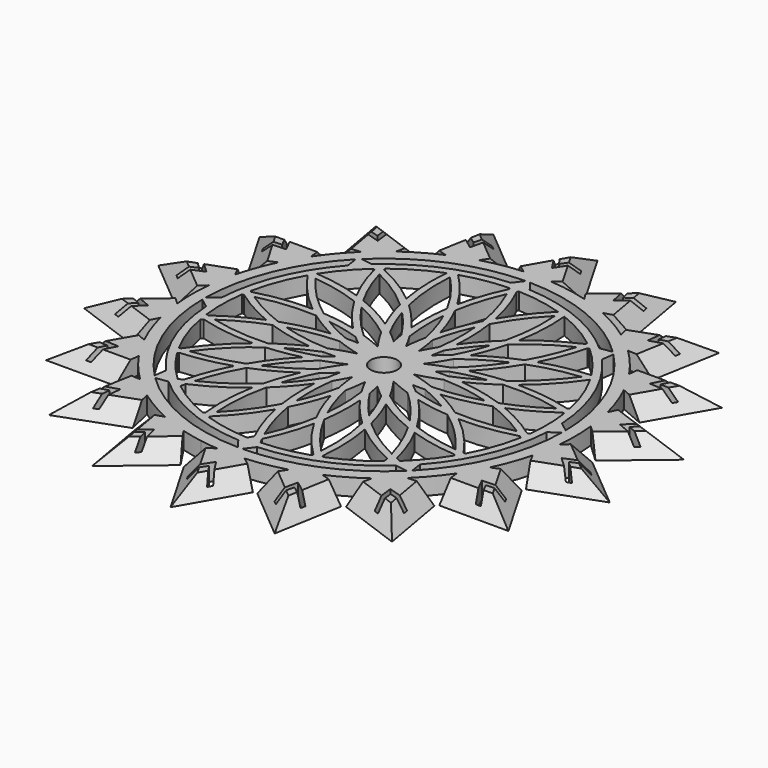
from build123d import *

# Parameters (mm, degrees)
F1_DEPTH      = 5.08
F2_T4_DEPTH   = 47.0360427955
F2_T9_DEPTH   = 47.0360427955
F2_T14_DEPTH  = 47.0360427955
F2_T19_DEPTH  = 47.0360427955
F2_T24_DEPTH  = 47.0360427955
F2_T29_DEPTH  = 47.0360427955
F2_T34_DEPTH  = 47.0360427955
F2_T39_DEPTH  = 47.0360427955
F2_T44_DEPTH  = 47.0360427955
F2_T49_DEPTH  = 47.0360427955
F2_T54_DEPTH  = 47.0360427955
F2_T59_DEPTH  = 47.0360427955
F2_T64_DEPTH  = 47.0360427955
F2_T69_DEPTH  = 47.0360427955
F2_T74_DEPTH  = 47.0360427955
F2_T79_DEPTH  = 47.0360427955
F2_T84_DEPTH  = 47.0360427955
F2_T89_DEPTH  = 47.0360427955
F2_T94_DEPTH  = 47.0360427955
F2_T99_DEPTH  = 47.0360427955
F2_T104_DEPTH = 47.0360427955
F2_T109_DEPTH = 47.0360427955
F2_T114_DEPTH = 47.0360427955
F2_T119_DEPTH = 47.0360427955
F2_T124_DEPTH = 47.0360427955
F2_T129_DEPTH = 47.0360427955
F2_T134_DEPTH = 47.0360427955
F2_T139_DEPTH = 47.0360427955
F2_T144_DEPTH = 47.0360427955
F2_T149_DEPTH = 47.0360427955
F2_T154_DEPTH = 47.0360427955
F2_T159_DEPTH = 47.0360427955
F2_T164_DEPTH = 47.0360427955
F2_T169_DEPTH = 47.0360427955
F2_T174_DEPTH = 47.0360427955
F2_T179_DEPTH = 47.0360427955
F4_DEPTH      = 5.08
F6_DEPTH      = 5.08
F7_R          = 55.2439698333
F7_R_2        = 49.2709923145
F8_DEPTH      = 5.08
F9_R          = 54.4459201536
F9_R_2        = 51.5980237821
F10_DEPTH     = 25.4
F12_DEPTH     = 5.08
F14_R         = 4.0270011847
F15_DEPTH     = 25.4


# Not quite as in the source:
# - a fillet or chamfer that OpenCascade refuses, or shapes differently, is made with other operations: its cross-section is extruded or revolved along the edge and cut away or added


with BuildPart() as f1:
    # F0 (on Top) → F1 (new body)
    with BuildSketch(Plane.XY):
        with BuildLine():
            ThreePointArc((15.9265090024, 55.862840854), (10.0864226386, 57.2064223286), (4.138989374, 57.941172272))
            Line((4.138989374, 57.941172272), (10.4434320733, 62.6353312958))
            Line((10.4434320733, 62.6353312958), (0, 80.7479918003))
            Line((0, 80.7479918003), (-10.4434320733, 62.6353312958))
            Line((-10.4434320733, 62.6353312958), (-4.140193851, 57.9410862184))
            ThreePointArc((-4.140193851, 57.9410862184), (-10.0876118404, 57.2062126403), (-15.9276702726, 55.8625097626))
            Line((-15.9276702726, 55.8625097626), (-11.6089289321, 62.4298227536))
            Line((-11.6089289321, 62.4298227536), (-27.6174397288, 75.878292038))
            Line((-27.6174397288, 75.878292038), (-31.236161042, 55.2860944846))
            Line((-31.236161042, 55.2860944846), (-23.7075282233, 53.0307814654))
            ThreePointArc((-23.7075282233, 53.0307814654), (-29.0449314541, 50.3060894337), (-34.073217817, 47.046004133))
            Line((-34.073217817, 47.046004133), (-32.2610817787, 54.6943562213))
            Line((-32.2610817787, 54.6943562213), (-51.9038086363, 61.8565504116))
            Line((-51.9038086363, 61.8565504116), (-48.2613479923, 41.2685387427))
            Line((-48.2613479923, 41.2685387427), (-40.415384806, 41.7241818167))
            ThreePointArc((-40.415384806, 41.7241818167), (-44.4990036769, 37.3383094027), (-48.1090324256, 32.5550560799))
            Line((-48.1090324256, 32.5550560799), (-49.02207204, 40.361943126))
            Line((-49.02207204, 40.361943126), (-69.9298122036, 40.3739959002))
            Line((-69.9298122036, 40.3739959002), (-59.4655041132, 22.2733881697))
            Line((-59.4655041132, 22.2733881697), (-52.2485495135, 25.3850300576))
            ThreePointArc((-52.2485495135, 25.3850300576), (-54.585839321, 19.8669782029), (-56.3421877099, 14.1374878021))
            Line((-56.3421877099, 14.1374878021), (-59.8702769245, 21.1612840109))
            Line((-59.8702769245, 21.1612840109), (-79.5212483651, 14.0217416264))
            Line((-79.5212483651, 14.0217416264), (-63.4972428207, 0.5917382633))
            Line((-63.4972428207, 0.5917382633), (-57.7797680432, 5.9840690304))
            ThreePointArc((-57.7797680432, 5.9840690304), (-58.0888171417, -0.0006037736), (-57.7796436342, -5.9852701517))
            Line((-57.7796436342, -5.9852701517), (-63.4972428207, -0.5917382633))
            Line((-63.4972428207, -0.5917382633), (-79.5212483651, -14.0217416264))
            Line((-79.5212483651, -14.0217416264), (-59.8702769245, -21.1612840109))
            Line((-59.8702769245, -21.1612840109), (-56.3418938084, -14.1386590373))
            ThreePointArc((-56.3418938084, -14.1386590373), (-54.5854263155, -19.868112926), (-52.2480217996, -25.3861161921))
            Line((-52.2480217996, -25.3861161921), (-59.4655041132, -22.2733881697))
            Line((-59.4655041132, -22.2733881697), (-69.9298122036, -40.3739959002))
            Line((-69.9298122036, -40.3739959002), (-49.02207204, -40.361943126))
            Line((-49.02207204, -40.361943126), (-48.1083556625, -32.5560561608))
            ThreePointArc((-48.1083556625, -32.5560561608), (-44.4982274806, -37.3392344374), (-40.4145174372, -41.7250219605))
            Line((-40.4145174372, -41.7250219605), (-48.2613479923, -41.2685387427))
            Line((-48.2613479923, -41.2685387427), (-51.9038086363, -61.8565504116))
            Line((-51.9038086363, -61.8565504116), (-32.2610817787, -54.6943562213))
            Line((-32.2610817787, -54.6943562213), (-34.0722398199, -47.046712435))
            ThreePointArc((-34.0722398199, -47.046712435), (-29.0438856876, -50.3066932073), (-23.7064258172, -53.0312742847))
            Line((-23.7064258172, -53.0312742847), (-31.236161042, -55.2860944846))
            Line((-31.236161042, -55.2860944846), (-27.6174397288, -75.878292038))
            Line((-27.6174397288, -75.878292038), (-11.6089289321, -62.4298227536))
            Line((-11.6089289321, -62.4298227536), (-15.9265090024, -55.862840854))
            ThreePointArc((-15.9265090024, -55.862840854), (-12.7601875814, -56.6699946195), (-9.5534900168, -57.2978315976))
            ThreePointArc((-9.5534900168, -57.2978315976), (-6.8578650316, -57.717343394), (-4.138989374, -57.941172272))
            Line((-4.138989374, -57.941172272), (-10.4434320733, -62.6353312958))
            Line((-10.4434320733, -62.6353312958), (0, -80.7479918003))
            Line((0, -80.7479918003), (10.4434320733, -62.6353312958))
            Line((10.4434320733, -62.6353312958), (4.140193851, -57.9410862184))
            ThreePointArc((4.140193851, -57.9410862184), (10.0876118404, -57.2062126403), (15.9276702726, -55.8625097626))
            Line((15.9276702726, -55.8625097626), (11.6089289321, -62.4298227536))
            Line((11.6089289321, -62.4298227536), (27.6174397288, -75.878292038))
            Line((27.6174397288, -75.878292038), (31.236161042, -55.2860944846))
            Line((31.236161042, -55.2860944846), (23.7075282233, -53.0307814654))
            ThreePointArc((23.7075282233, -53.0307814654), (29.0449314541, -50.3060894337), (34.073217817, -47.046004133))
            Line((34.073217817, -47.046004133), (32.2610817787, -54.6943562213))
            Line((32.2610817787, -54.6943562213), (51.9038086363, -61.8565504116))
            Line((51.9038086363, -61.8565504116), (48.2613479923, -41.2685387427))
            Line((48.2613479923, -41.2685387427), (40.415384806, -41.7241818167))
            ThreePointArc((40.415384806, -41.7241818167), (44.4990036769, -37.3383094027), (48.1090324256, -32.5550560799))
            Line((48.1090324256, -32.5550560799), (49.02207204, -40.361943126))
            Line((49.02207204, -40.361943126), (69.9298122036, -40.3739959002))
            Line((69.9298122036, -40.3739959002), (59.4655041132, -22.2733881697))
            Line((59.4655041132, -22.2733881697), (52.2485495135, -25.3850300576))
            ThreePointArc((52.2485495135, -25.3850300576), (54.585839321, -19.8669782029), (56.3421877099, -14.1374878021))
            Line((56.3421877099, -14.1374878021), (59.8702769245, -21.1612840109))
            Line((59.8702769245, -21.1612840109), (79.5212483651, -14.0217416264))
            Line((79.5212483651, -14.0217416264), (63.4972428207, -0.5917382633))
            Line((63.4972428207, -0.5917382633), (57.7797680432, -5.9840690304))
            ThreePointArc((57.7797680432, -5.9840690304), (58.0888171417, 0.0006037736), (57.7796436342, 5.9852701517))
            Line((57.7796436342, 5.9852701517), (63.4972428207, 0.5917382633))
            Line((63.4972428207, 0.5917382633), (79.5212483651, 14.0217416264))
            Line((79.5212483651, 14.0217416264), (59.8702769245, 21.1612840109))
            Line((59.8702769245, 21.1612840109), (56.3418938084, 14.1386590373))
            ThreePointArc((56.3418938084, 14.1386590373), (54.5854263155, 19.868112926), (52.2480217996, 25.3861161921))
            Line((52.2480217996, 25.3861161921), (59.4655041132, 22.2733881697))
            Line((59.4655041132, 22.2733881697), (69.9298122036, 40.3739959002))
            Line((69.9298122036, 40.3739959002), (49.02207204, 40.361943126))
            Line((49.02207204, 40.361943126), (48.1083556625, 32.5560561608))
            ThreePointArc((48.1083556625, 32.5560561608), (44.4982274806, 37.3392344374), (40.4145174372, 41.7250219605))
            Line((40.4145174372, 41.7250219605), (48.2613479923, 41.2685387427))
            Line((48.2613479923, 41.2685387427), (51.9038086363, 61.8565504116))
            Line((51.9038086363, 61.8565504116), (32.2610817787, 54.6943562213))
            Line((32.2610817787, 54.6943562213), (34.0722398199, 47.046712435))
            ThreePointArc((34.0722398199, 47.046712435), (29.0438856876, 50.3066932073), (23.7064258172, 53.0312742847))
            Line((23.7064258172, 53.0312742847), (31.236161042, 55.2860944846))
            Line((31.236161042, 55.2860944846), (27.6174397288, 75.878292038))
            Line((27.6174397288, 75.878292038), (11.6089289321, 62.4298227536))
            Line((11.6089289321, 62.4298227536), (15.9265090024, 55.862840854))
        make_face()
        Polygon((-40.8170132151, -48.6438221381), (-41.6786948496, -55.6460012024), (-43.1171047598, -56.1704788463), (-42.4937358465, -50.6420623579), (-47.8299146071, -52.2159618416), (-47.5631825433, -50.708329749), align=None, mode=Mode.SUBTRACT)
        Polygon((-21.7182791012, -59.6704814199), (-20.1331086874, -66.5450898922), (-21.3053899468, -67.5299028276), (-22.6104445787, -62.1216859237), (-27.0865070562, -65.425748279), (-27.3515014484, -63.917809788), align=None, mode=Mode.SUBTRACT)
        Polygon((-54.9926131403, -31.75), (-58.1972153009, -38.03518352), (-59.7282603981, -38.0360661281), (-57.2516554306, -33.0542586744), (-62.8043285621, -32.7081597806), (-62.0380418656, -31.382676767), align=None, mode=Mode.SUBTRACT)
        Polygon((-62.5352923163, -11.0266592818), (-67.6962926875, -15.8367613656), (-69.1353063372, -15.3139424824), (-65.1041804252, -11.4796235659), (-70.2036135993, -9.255270929), (-69.0301977549, -8.271809808), align=None, mode=Mode.SUBTRACT)
        Polygon((3.0760693279, -70.7442238927), (0, -66.1085173488), (-3.076067, -70.7442238927), (-3.8408256137, -69.4178586401), (0, -63.5), (3.8408275155, -69.4178586401), align=None, mode=Mode.SUBTRACT)
        Polygon((27.0865092437, -65.4257474828), (22.6104445787, -62.1216859237), (21.3053921343, -67.5299020314), (20.1331104745, -66.5450892418), (21.7182791012, -59.6704814199), (27.3515032355, -63.9178091375), align=None, mode=Mode.SUBTRACT)
        Polygon((47.8299163904, -52.2159603452), (42.4937358465, -50.6420623579), (43.1171065431, -56.1704773499), (41.6786963064, -55.64599998), (40.8170132151, -48.6438221381), (47.563184, -50.7083285266), align=None, mode=Mode.SUBTRACT)
        with BuildLine():
            ThreePointArc((53.4287791534, 0), (-37.7798520499, -37.7798520499), (0, 53.4287791534))
            ThreePointArc((0, 53.4287791534), (37.7798520499, 37.7798520499), (53.4287791534, 0))
        make_face(mode=Mode.SUBTRACT)
        Polygon((62.804329726, -32.7081577646), (57.2516554306, -33.0542586744), (59.7282615621, -38.0360641121), (58.1972162518, -38.0351818731), (54.9926131403, -31.75), (62.0380428164, -31.3826751201), align=None, mode=Mode.SUBTRACT)
        Polygon((70.2036140035, -9.2552686365), (65.1041804252, -11.4796235659), (69.1353067414, -15.3139401898), (67.6962930177, -15.8367594928), (62.5352923163, -11.0266592819), (69.0301980851, -8.2718079352), align=None, mode=Mode.SUBTRACT)
        Polygon((-62.5352923163, 11.0266592819), (-69.0301980851, 8.2718079352), (-70.2036140035, 9.2552686365), (-65.1041804252, 11.4796235659), (-69.1353067414, 15.3139401898), (-67.6962930177, 15.8367594928), align=None, mode=Mode.SUBTRACT)
        Polygon((-54.9926131403, 31.75), (-62.0380428164, 31.3826751201), (-62.804329726, 32.7081577646), (-57.2516554306, 33.0542586744), (-59.7282615621, 38.0360641121), (-58.1972162518, 38.0351818731), align=None, mode=Mode.SUBTRACT)
        Polygon((-40.8170132151, 48.6438221381), (-47.563184, 50.7083285266), (-47.8299163904, 52.2159603452), (-42.4937358465, 50.6420623579), (-43.1171065431, 56.1704773499), (-41.6786963064, 55.64599998), align=None, mode=Mode.SUBTRACT)
        Polygon((-21.7182791012, 59.6704814199), (-27.3515032355, 63.9178091376), (-27.0865092437, 65.4257474828), (-22.6104445787, 62.1216859237), (-21.3053921343, 67.5299020314), (-20.1331104745, 66.5450892418), align=None, mode=Mode.SUBTRACT)
        Polygon((3.8408256138, 69.4178586401), (0, 63.5), (-3.8408275155, 69.4178586401), (-3.0760693279, 70.7442238927), (0, 66.1085173488), (3.076067, 70.7442238927), align=None, mode=Mode.SUBTRACT)
        Polygon((69.1353063372, 15.3139424824), (65.1041804252, 11.4796235659), (70.2036135993, 9.255270929), (69.0301977548, 8.271809808), (62.5352923163, 11.0266592818), (67.6962926875, 15.8367613656), align=None, mode=Mode.SUBTRACT)
        Polygon((59.7282603981, 38.0360661281), (57.2516554306, 33.0542586744), (62.8043285621, 32.7081597806), (62.0380418655, 31.382676767), (54.9926131403, 31.75), (58.1972153009, 38.03518352), align=None, mode=Mode.SUBTRACT)
        Polygon((21.3053899468, 67.5299028276), (22.6104445787, 62.1216859237), (27.0865070562, 65.425748279), (27.3515014484, 63.917809788), (21.7182791012, 59.6704814199), (20.1331086874, 66.5450898922), align=None, mode=Mode.SUBTRACT)
        Polygon((43.1171047598, 56.1704788463), (42.4937358465, 50.6420623579), (47.8299146071, 52.2159618416), (47.5631825432, 50.708329749), (40.8170132151, 48.6438221381), (41.6786948496, 55.6460012024), align=None, mode=Mode.SUBTRACT)
    extrude(amount=F1_DEPTH)

    # F2: chamfer of 5.08 on 36 edges, made by hand


with BuildPart() as f2_tool2:
    # F2_s3 → F2_t4 (new body)
    with BuildSketch(Plane(origin=(-6.2684927358, -35.4309391934, 0), x_dir=(0, 0, 1), z_dir=(-0.174215865, -0.9847074857, 0))):
        Polygon((5.08, 35.2536764612), (0, 40.3336764612), (5.08, 40.3336764612), align=None)
    extrude(amount=F2_T4_DEPTH)

    split(bisect_by=Plane(origin=(-2.5554446187, -43.9274438504, 0), x_dir=(0, 0, 1), z_dir=(-0.0580760277, -0.9983121631, 0)), keep=Keep.TOP)


with BuildPart() as f1_1:
    add(f1.part)

    # F2_t1: cut F2_tool2
    add(f2_tool2.part, mode=Mode.SUBTRACT)


with BuildPart() as f2_tool7:
    # F2_s8 → F2_t9 (new body)
    with BuildSketch(Plane(origin=(-77.9942923576, -28.4385295204, 0), x_dir=(0, 0, 1), z_dir=(0.9394952989, 0.342561795, 0))):
        Polygon((5.08, 35.2536764612), (0, 40.3336764612), (5.08, 40.3336764612), align=None)
    extrude(amount=F2_T9_DEPTH)

    split(bisect_by=Plane(origin=(-42.8128872524, -10.1391889033, 0), x_dir=(0, 0, 1), z_dir=(-0.9730838832, -0.2304512016, 0)), keep=Keep.TOP)


with BuildPart() as f1_2:
    add(f1_1.part)

    # F2_t6: cut F2_tool7
    add(f2_tool7.part, mode=Mode.SUBTRACT)


with BuildPart() as f2_tool12:
    # F2_s13 → F2_t14 (new body)
    with BuildSketch(Plane(origin=(6.2276385338, -35.4381428915, 0), x_dir=(0, 0, 1), z_dir=(0.1730804326, -0.9849076931, 0))):
        Polygon((5.08, 35.2536764612), (0, 40.3336764612), (5.08, 40.3336764612), align=None)
    extrude(amount=F2_T14_DEPTH)

    split(bisect_by=Plane(origin=(12.6227381906, -42.1523083709, 0), x_dir=(0, 0, 1), z_dir=(0.2868692545, -0.9579697442, 0)), keep=Keep.TOP)


with BuildPart() as f1_3:
    add(f1_2.part)

    # F2_t11: cut F2_tool12
    add(f2_tool12.part, mode=Mode.SUBTRACT)


with BuildPart() as f2_tool17:
    # F2_s18 → F2_t19 (new body)
    with BuildSketch(Plane(origin=(-63.5641110493, -53.399095387, 0), x_dir=(0, 0, 1), z_dir=(0.7656737654, 0.6432291077, 0))):
        Polygon((5.08, 35.2536764612), (0, 40.3336764612), (5.08, 40.3336764612), align=None)
    extrude(amount=F2_T19_DEPTH)

    split(bisect_by=Plane(origin=(-36.7631473837, -24.1705908274, 0), x_dir=(0, 0, 1), z_dir=(-0.8355807914, -0.5493675828, 0)), keep=Keep.TOP)


with BuildPart() as f1_4:
    add(f1_3.part)

    # F2_t16: cut F2_tool17
    add(f2_tool17.part, mode=Mode.SUBTRACT)


with BuildPart() as f2_tool22:
    # F2_s23 → F2_t24 (new body)
    with BuildSketch(Plane(origin=(17.9726246861, -31.1709835456, 0), x_dir=(0, 0, 1), z_dir=(0.4995006756, -0.866313497, 0))):
        Polygon((5.08, 35.2536764612), (0, 40.3336764612), (5.08, 40.3336764612), align=None)
    extrude(amount=F2_T24_DEPTH)

    split(bisect_by=Plane(origin=(26.2784324824, -35.2929824001, 0), x_dir=(0, 0, 1), z_dir=(0.5972138708, -0.8020820361, 0)), keep=Keep.TOP)


with BuildPart() as f1_5:
    add(f1_4.part)

    # F2_t21: cut F2_tool22
    add(f2_tool22.part, mode=Mode.SUBTRACT)


with BuildPart() as f2_tool27:
    # F2_s28 → F2_t29 (new body)
    with BuildSketch(Plane(origin=(-41.4671598421, -71.9189422632, 0), x_dir=(0, 0, 1), z_dir=(0.4995006756, 0.866313497, 0))):
        Polygon((5.08, 35.2536764613), (0, 40.3336764613), (5.08, 40.3336764613), align=None)
    extrude(amount=F2_T29_DEPTH)

    split(bisect_by=Plane(origin=(-26.2792293743, -35.2866627778, 0), x_dir=(0, 0, 1), z_dir=(-0.5972943244, -0.8020221257, 0)), keep=Keep.TOP)


with BuildPart() as f1_6:
    add(f1_5.part)

    # F2_t26: cut F2_tool27
    add(f2_tool27.part, mode=Mode.SUBTRACT)


with BuildPart() as f2_tool32:
    # F2_s33 → F2_t34 (new body)
    with BuildSketch(Plane(origin=(27.5498470535, -23.1441435493, 0), x_dir=(0, 0, 1), z_dir=(0.7656737654, -0.6432291077, 0))):
        Polygon((5.08, 35.2536764612), (0, 40.3336764612), (5.08, 40.3336764612), align=None)
    extrude(amount=F2_T34_DEPTH)

    split(bisect_by=Plane(origin=(36.7645599884, -24.1768018828, 0), x_dir=(0, 0, 1), z_dir=(0.8355256803, -0.5494513969, 0)), keep=Keep.TOP)


with BuildPart() as f1_7:
    add(f1_6.part)

    # F2_t31: cut F2_tool32
    add(f2_tool32.part, mode=Mode.SUBTRACT)


with BuildPart() as f2_tool37:
    # F2_s38 → F2_t39 (new body)
    with BuildSketch(Plane(origin=(-14.3686571678, -81.7643032921, 0), x_dir=(0, 0, 1), z_dir=(0.1730804326, 0.9849076931, 0))):
        Polygon((5.08, 35.2536764612), (0, 40.3336764612), (5.08, 40.3336764612), align=None)
    extrude(amount=F2_T39_DEPTH)

    split(bisect_by=Plane(origin=(-12.6256484622, -42.1466424216, 0), x_dir=(0, 0, 1), z_dir=(-0.2869653467, -0.9579409636, 0)), keep=Keep.TOP)


with BuildPart() as f1_8:
    add(f1_7.part)

    # F2_t36: cut F2_tool37
    add(f2_tool37.part, mode=Mode.SUBTRACT)


with BuildPart() as f2_tool42:
    # F2_s43 → F2_t44 (new body)
    with BuildSketch(Plane(origin=(33.8041512739, -12.3257782699, 0), x_dir=(0, 0, 1), z_dir=(0.9394952989, -0.342561795, 0))):
        Polygon((5.08, 35.2536764612), (0, 40.3336764612), (5.08, 40.3336764612), align=None)
    extrude(amount=F2_T44_DEPTH)

    split(bisect_by=Plane(origin=(42.8163389727, -10.144542247, 0), x_dir=(0, 0, 1), z_dir=(0.9730607618, -0.2305488102, 0)), keep=Keep.TOP)


with BuildPart() as f1_9:
    add(f1_8.part)

    # F2_t41: cut F2_tool42
    add(f2_tool42.part, mode=Mode.SUBTRACT)


with BuildPart() as f2_tool47:
    # F2_s48 → F2_t49 (new body)
    with BuildSketch(Plane(origin=(14.4629176196, -81.7476826312, 0), x_dir=(0, 0, 1), z_dir=(-0.174215865, 0.9847074857, 0))):
        Polygon((5.08, 35.2536764612), (0, 40.3336764612), (5.08, 40.3336764612), align=None)
    extrude(amount=F2_T49_DEPTH)

    split(bisect_by=Plane(origin=(2.5507719892, -43.9231149711, 0), x_dir=(0, 0, 1), z_dir=(0.057975887, -0.9983179837, 0)), keep=Keep.TOP)


with BuildPart() as f1_10:
    add(f1_9.part)

    # F2_t46: cut F2_tool47
    add(f2_tool47.part, mode=Mode.SUBTRACT)


with BuildPart() as f2_tool52:
    # F2_s53 → F2_t54 (new body)
    with BuildSketch(Plane(origin=(35.9811759544, -0.0207422219, 0), x_dir=(0, 0, 1), z_dir=(0.9999998338, -0.0005764742, 0))):
        Polygon((5.08, 35.2536764612), (0, 40.3336764612), (5.08, 40.3336764612), align=None)
    extrude(amount=F2_T54_DEPTH)

    split(bisect_by=Plane(origin=(43.703835575, 5.1112989013, 0), x_dir=(0, 0, 1), z_dir=(0.9932303545, 0.1161613655, 0)), keep=Keep.TOP)


with BuildPart() as f1_11:
    add(f1_10.part)

    # F2_t51: cut F2_tool52
    add(f2_tool52.part, mode=Mode.SUBTRACT)


with BuildPart() as f2_tool57:
    # F2_s58 → F2_t59 (new body)
    with BuildSketch(Plane(origin=(41.5500510922, -71.8710849777, 0), x_dir=(0, 0, 1), z_dir=(-0.5004991582, 0.8657370228, 0))):
        Polygon((5.08, 35.2536764612), (0, 40.3336764612), (5.08, 40.3336764612), align=None)
    extrude(amount=F2_T59_DEPTH)

    split(bisect_by=Plane(origin=(17.4195316933, -40.401811619, 0), x_dir=(0, 0, 1), z_dir=(0.395924373, -0.9182831213, 0)), keep=Keep.TOP)


with BuildPart() as f1_12:
    add(f1_11.part)

    # F2_t56: cut F2_tool57
    add(f2_tool57.part, mode=Mode.SUBTRACT)


with BuildPart() as f2_tool62:
    # F2_s63 → F2_t64 (new body)
    with BuildSketch(Plane(origin=(33.8183397893, 12.2867956441, 0), x_dir=(0, 0, 1), z_dir=(0.9398896304, 0.341478378, 0))):
        Polygon((5.08, 35.2536764612), (0, 40.3336764612), (5.08, 40.3336764612), align=None)
    extrude(amount=F2_T64_DEPTH)

    split(bisect_by=Plane(origin=(39.3200046071, 19.7506419674, 0), x_dir=(0, 0, 1), z_dir=(0.893601708, 0.4488607662, 0)), keep=Keep.TOP)


with BuildPart() as f1_13:
    add(f1_12.part)

    # F2_t61: cut F2_tool62
    add(f2_tool62.part, mode=Mode.SUBTRACT)


with BuildPart() as f2_tool67:
    # F2_s68 → F2_t69 (new body)
    with BuildSketch(Plane(origin=(63.6256351897, -53.3257737717, 0), x_dir=(0, 0, 1), z_dir=(-0.7664148663, 0.642345898, 0))):
        Polygon((5.08, 35.2536764612), (0, 40.3336764612), (5.08, 40.3336764612), align=None)
    extrude(amount=F2_T69_DEPTH)

    split(bisect_by=Plane(origin=(30.1872387902, -32.0074535183, 0), x_dir=(0, 0, 1), z_dir=(0.6861185365, -0.7274897621, 0)), keep=Keep.TOP)


with BuildPart() as f1_14:
    add(f1_13.part)

    # F2_t66: cut F2_tool67
    add(f2_tool67.part, mode=Mode.SUBTRACT)


with BuildPart() as f2_tool72:
    # F2_s73 → F2_t74 (new body)
    with BuildSketch(Plane(origin=(27.57651274, 23.1123646216, 0), x_dir=(0, 0, 1), z_dir=(0.7664148663, 0.642345898, 0))):
        Polygon((5.08, 35.2536764612), (0, 40.3336764612), (5.08, 40.3336764612), align=None)
    extrude(amount=F2_T74_DEPTH)

    split(bisect_by=Plane(origin=(30.193600782, 32.0077661239, 0), x_dir=(0, 0, 1), z_dir=(0.6861915073, 0.727420934, 0)), keep=Keep.TOP)


with BuildPart() as f1_15:
    add(f1_14.part)

    # F2_t71: cut F2_tool72
    add(f2_tool72.part, mode=Mode.SUBTRACT)


with BuildPart() as f2_tool77:
    # F2_s78 → F2_t79 (new body)
    with BuildSketch(Plane(origin=(78.0270286689, -28.3485872441, 0), x_dir=(0, 0, 1), z_dir=(-0.9398896304, 0.341478378, 0))):
        Polygon((5.08, 35.2536764612), (0, 40.3336764612), (5.08, 40.3336764612), align=None)
    extrude(amount=F2_T79_DEPTH)

    split(bisect_by=Plane(origin=(39.3139193729, -19.7525241437, 0), x_dir=(0, 0, 1), z_dir=(0.8935566784, -0.4489504009, 0)), keep=Keep.TOP)


with BuildPart() as f1_16:
    add(f1_15.part)

    # F2_t76: cut F2_tool77
    add(f2_tool77.part, mode=Mode.SUBTRACT)


with BuildPart() as f2_tool82:
    # F2_s83 → F2_t84 (new body)
    with BuildSketch(Plane(origin=(41.4671598421, 71.9189422633, 0), x_dir=(0, 0, 1), z_dir=(-0.4995006756, -0.866313497, 0))):
        Polygon((5.08, 35.2536764612), (0, 40.3336764612), (5.08, 40.3336764612), align=None)
    extrude(amount=F2_T84_DEPTH)

    split(bisect_by=Plane(origin=(26.2792293743, 35.2866627779, 0), x_dir=(0, 0, 1), z_dir=(0.5972943244, 0.8020221257, 0)), keep=Keep.TOP)


with BuildPart() as f1_17:
    add(f1_16.part)

    # F2_t81: cut F2_tool82
    add(f2_tool82.part, mode=Mode.SUBTRACT)


with BuildPart() as f2_tool87:
    # F2_s88 → F2_t89 (new body)
    with BuildSketch(Plane(origin=(-27.5498470535, 23.1441435493, 0), x_dir=(0, 0, 1), z_dir=(-0.7656737654, 0.6432291077, 0))):
        Polygon((5.08, 35.2536764612), (0, 40.3336764612), (5.08, 40.3336764612), align=None)
    extrude(amount=F2_T89_DEPTH)

    split(bisect_by=Plane(origin=(-36.7645599884, 24.1768018829, 0), x_dir=(0, 0, 1), z_dir=(-0.8355256803, 0.5494513969, 0)), keep=Keep.TOP)


with BuildPart() as f1_18:
    add(f1_17.part)

    # F2_t86: cut F2_tool87
    add(f2_tool87.part, mode=Mode.SUBTRACT)


with BuildPart() as f2_tool92:
    # F2_s93 → F2_t94 (new body)
    with BuildSketch(Plane(origin=(14.3686571679, 81.764303292, 0), x_dir=(0, 0, 1), z_dir=(-0.1730804326, -0.9849076931, 0))):
        Polygon((5.08, 35.2536764612), (0, 40.3336764612), (5.08, 40.3336764612), align=None)
    extrude(amount=F2_T94_DEPTH)

    split(bisect_by=Plane(origin=(12.6256484622, 42.1466424216, 0), x_dir=(0, 0, 1), z_dir=(0.2869653467, 0.9579409636, 0)), keep=Keep.TOP)


with BuildPart() as f1_19:
    add(f1_18.part)

    # F2_t91: cut F2_tool92
    add(f2_tool92.part, mode=Mode.SUBTRACT)


with BuildPart() as f2_tool97:
    # F2_s98 → F2_t99 (new body)
    with BuildSketch(Plane(origin=(-33.8041512739, 12.3257782699, 0), x_dir=(0, 0, 1), z_dir=(-0.9394952989, 0.342561795, 0))):
        Polygon((5.08, 35.2536764612), (0, 40.3336764612), (5.08, 40.3336764612), align=None)
    extrude(amount=F2_T99_DEPTH)

    split(bisect_by=Plane(origin=(-42.8163389727, 10.144542247, 0), x_dir=(0, 0, 1), z_dir=(-0.9730607618, 0.2305488102, 0)), keep=Keep.TOP)


with BuildPart() as f1_20:
    add(f1_19.part)

    # F2_t96: cut F2_tool97
    add(f2_tool97.part, mode=Mode.SUBTRACT)


with BuildPart() as f2_tool102:
    # F2_s103 → F2_t104 (new body)
    with BuildSketch(Plane(origin=(-14.4629176196, 81.7476826312, 0), x_dir=(0, 0, 1), z_dir=(0.174215865, -0.9847074857, 0))):
        Polygon((5.08, 35.2536764612), (0, 40.3336764612), (5.08, 40.3336764612), align=None)
    extrude(amount=F2_T104_DEPTH)

    split(bisect_by=Plane(origin=(-2.5507719892, 43.9231149711, 0), x_dir=(0, 0, 1), z_dir=(-0.057975887, 0.9983179837, 0)), keep=Keep.TOP)


with BuildPart() as f1_21:
    add(f1_20.part)

    # F2_t101: cut F2_tool102
    add(f2_tool102.part, mode=Mode.SUBTRACT)


with BuildPart() as f2_tool107:
    # F2_s108 → F2_t109 (new body)
    with BuildSketch(Plane(origin=(-35.9811759544, 0.0207422219, 0), x_dir=(0, 0, 1), z_dir=(-0.9999998338, 0.0005764742, 0))):
        Polygon((5.08, 35.2536764612), (0, 40.3336764612), (5.08, 40.3336764612), align=None)
    extrude(amount=F2_T109_DEPTH)

    split(bisect_by=Plane(origin=(-43.703835575, -5.1112989013, 0), x_dir=(0, 0, 1), z_dir=(-0.9932303545, -0.1161613655, 0)), keep=Keep.TOP)


with BuildPart() as f1_22:
    add(f1_21.part)

    # F2_t106: cut F2_tool107
    add(f2_tool107.part, mode=Mode.SUBTRACT)


with BuildPart() as f2_tool112:
    # F2_s113 → F2_t114 (new body)
    with BuildSketch(Plane(origin=(-41.5500510923, 71.8710849777, 0), x_dir=(0, 0, 1), z_dir=(0.5004991582, -0.8657370228, 0))):
        Polygon((5.08, 35.2536764612), (0, 40.3336764612), (5.08, 40.3336764612), align=None)
    extrude(amount=F2_T114_DEPTH)

    split(bisect_by=Plane(origin=(-17.4195316933, 40.401811619, 0), x_dir=(0, 0, 1), z_dir=(-0.395924373, 0.9182831213, 0)), keep=Keep.TOP)


with BuildPart() as f1_23:
    add(f1_22.part)

    # F2_t111: cut F2_tool112
    add(f2_tool112.part, mode=Mode.SUBTRACT)


with BuildPart() as f2_tool117:
    # F2_s118 → F2_t119 (new body)
    with BuildSketch(Plane(origin=(-33.8183397893, -12.2867956441, 0), x_dir=(0, 0, 1), z_dir=(-0.9398896304, -0.341478378, 0))):
        Polygon((5.08, 35.2536764612), (0, 40.3336764612), (5.08, 40.3336764612), align=None)
    extrude(amount=F2_T119_DEPTH)

    split(bisect_by=Plane(origin=(-39.320004607, -19.7506419675, 0), x_dir=(0, 0, 1), z_dir=(-0.893601708, -0.4488607662, 0)), keep=Keep.TOP)


with BuildPart() as f1_24:
    add(f1_23.part)

    # F2_t116: cut F2_tool117
    add(f2_tool117.part, mode=Mode.SUBTRACT)


with BuildPart() as f2_tool122:
    # F2_s123 → F2_t124 (new body)
    with BuildSketch(Plane(origin=(-63.6256351897, 53.3257737716, 0), x_dir=(0, 0, 1), z_dir=(0.7664148663, -0.642345898, 0))):
        Polygon((5.08, 35.2536764612), (0, 40.3336764612), (5.08, 40.3336764612), align=None)
    extrude(amount=F2_T124_DEPTH)

    split(bisect_by=Plane(origin=(-30.1872387902, 32.0074535183, 0), x_dir=(0, 0, 1), z_dir=(-0.6861185365, 0.7274897621, 0)), keep=Keep.TOP)


with BuildPart() as f1_25:
    add(f1_24.part)

    # F2_t121: cut F2_tool122
    add(f2_tool122.part, mode=Mode.SUBTRACT)


with BuildPart() as f2_tool127:
    # F2_s128 → F2_t129 (new body)
    with BuildSketch(Plane(origin=(-27.57651274, -23.1123646216, 0), x_dir=(0, 0, 1), z_dir=(-0.7664148663, -0.642345898, 0))):
        Polygon((5.08, 35.2536764612), (0, 40.3336764612), (5.08, 40.3336764612), align=None)
    extrude(amount=F2_T129_DEPTH)

    split(bisect_by=Plane(origin=(-30.193600782, -32.0077661239, 0), x_dir=(0, 0, 1), z_dir=(-0.6861915073, -0.727420934, 0)), keep=Keep.TOP)


with BuildPart() as f1_26:
    add(f1_25.part)

    # F2_t126: cut F2_tool127
    add(f2_tool127.part, mode=Mode.SUBTRACT)


with BuildPart() as f2_tool132:
    # F2_s133 → F2_t134 (new body)
    with BuildSketch(Plane(origin=(-78.0270286689, 28.3485872441, 0), x_dir=(0, 0, 1), z_dir=(0.9398896304, -0.341478378, 0))):
        Polygon((5.08, 35.2536764612), (0, 40.3336764612), (5.08, 40.3336764612), align=None)
    extrude(amount=F2_T134_DEPTH)

    split(bisect_by=Plane(origin=(-39.3139193729, 19.7525241437, 0), x_dir=(0, 0, 1), z_dir=(-0.8935566784, 0.4489504009, 0)), keep=Keep.TOP)


with BuildPart() as f1_27:
    add(f1_26.part)

    # F2_t131: cut F2_tool132
    add(f2_tool132.part, mode=Mode.SUBTRACT)


with BuildPart() as f2_tool137:
    # F2_s138 → F2_t139 (new body)
    with BuildSketch(Plane(origin=(-18.0085512683, -31.1502413236, 0), x_dir=(0, 0, 1), z_dir=(-0.5004991582, -0.8657370228, 0))):
        Polygon((5.08, 35.2536764612), (0, 40.3336764612), (5.08, 40.3336764612), align=None)
    extrude(amount=F2_T139_DEPTH)

    split(bisect_by=Plane(origin=(-17.4254030926, -40.4042813014, 0), x_dir=(0, 0, 1), z_dir=(-0.3960164838, -0.9182434016, 0)), keep=Keep.TOP)


with BuildPart() as f1_28:
    add(f1_27.part)

    # F2_t136: cut F2_tool137
    add(f2_tool137.part, mode=Mode.SUBTRACT)


with BuildPart() as f2_tool142:
    # F2_s143 → F2_t144 (new body)
    with BuildSketch(Plane(origin=(-83.0172109344, -0.0478572856, 0), x_dir=(0, 0, 1), z_dir=(0.9999998338, 0.0005764742, 0))):
        Polygon((5.08, 35.2536764612), (0, 40.3336764612), (5.08, 40.3336764612), align=None)
    extrude(amount=F2_T144_DEPTH)

    split(bisect_by=Plane(origin=(-43.6987610676, 5.1151488411, 0), x_dir=(0, 0, 1), z_dir=(-0.9932186974, 0.1162609956, 0)), keep=Keep.TOP)


with BuildPart() as f1_29:
    add(f1_28.part)

    # F2_t141: cut F2_tool142
    add(f2_tool142.part, mode=Mode.SUBTRACT)


with BuildPart() as f2_tool147:
    # F2_s148 → F2_t149 (new body)
    with BuildSketch(Plane(origin=(-17.9726246861, 31.1709835456, 0), x_dir=(0, 0, 1), z_dir=(-0.4995006756, 0.866313497, 0))):
        Polygon((5.08, 35.2536764612), (0, 40.3336764612), (5.08, 40.3336764612), align=None)
    extrude(amount=F2_T149_DEPTH)

    split(bisect_by=Plane(origin=(-26.2784324824, 35.2929824001, 0), x_dir=(0, 0, 1), z_dir=(-0.5972138708, 0.8020820361, 0)), keep=Keep.TOP)


with BuildPart() as f1_30:
    add(f1_29.part)

    # F2_t146: cut F2_tool147
    add(f2_tool147.part, mode=Mode.SUBTRACT)


with BuildPart() as f2_tool152:
    # F2_s153 → F2_t154 (new body)
    with BuildSketch(Plane(origin=(63.5641110493, 53.399095387, 0), x_dir=(0, 0, 1), z_dir=(-0.7656737654, -0.6432291077, 0))):
        Polygon((5.08, 35.2536764612), (0, 40.3336764612), (5.08, 40.3336764612), align=None)
    extrude(amount=F2_T154_DEPTH)

    split(bisect_by=Plane(origin=(36.7631473837, 24.1705908274, 0), x_dir=(0, 0, 1), z_dir=(0.8355807914, 0.5493675828, 0)), keep=Keep.TOP)


with BuildPart() as f1_31:
    add(f1_30.part)

    # F2_t151: cut F2_tool152
    add(f2_tool152.part, mode=Mode.SUBTRACT)


with BuildPart() as f2_tool157:
    # F2_s158 → F2_t159 (new body)
    with BuildSketch(Plane(origin=(-6.2276385338, 35.4381428915, 0), x_dir=(0, 0, 1), z_dir=(-0.1730804326, 0.9849076931, 0))):
        Polygon((0, 40.3336764612), (5.08, 35.2536764612), (5.08, 40.3336764612), align=None)
    extrude(amount=F2_T159_DEPTH)

    split(bisect_by=Plane(origin=(-12.6227381906, 42.1523083709, 0), x_dir=(0, 0, 1), z_dir=(-0.2868692545, 0.9579697442, 0)), keep=Keep.TOP)


with BuildPart() as f1_32:
    add(f1_31.part)

    # F2_t156: cut F2_tool157
    add(f2_tool157.part, mode=Mode.SUBTRACT)


with BuildPart() as f2_tool162:
    # F2_s163 → F2_t164 (new body)
    with BuildSketch(Plane(origin=(77.9942923576, 28.4385295204, 0), x_dir=(0, 0, 1), z_dir=(-0.9394952989, -0.342561795, 0))):
        Polygon((5.08, 35.2536764612), (0, 40.3336764612), (5.08, 40.3336764612), align=None)
    extrude(amount=F2_T164_DEPTH)

    split(bisect_by=Plane(origin=(42.8128872524, 10.1391889033, 0), x_dir=(0, 0, 1), z_dir=(0.9730838832, 0.2304512016, 0)), keep=Keep.TOP)


with BuildPart() as f1_33:
    add(f1_32.part)

    # F2_t161: cut F2_tool162
    add(f2_tool162.part, mode=Mode.SUBTRACT)


with BuildPart() as f2_tool167:
    # F2_s168 → F2_t169 (new body)
    with BuildSketch(Plane(origin=(6.2684927358, 35.4309391934, 0), x_dir=(0, 0, 1), z_dir=(0.174215865, 0.9847074857, 0))):
        Polygon((5.08, 35.2536764612), (0, 40.3336764612), (5.08, 40.3336764612), align=None)
    extrude(amount=F2_T169_DEPTH)

    split(bisect_by=Plane(origin=(2.5554446187, 43.9274438504, 0), x_dir=(0, 0, 1), z_dir=(0.0580760277, 0.9983121631, 0)), keep=Keep.TOP)


with BuildPart() as f1_34:
    add(f1_33.part)

    # F2_t166: cut F2_tool167
    add(f2_tool167.part, mode=Mode.SUBTRACT)


with BuildPart() as f2_tool172:
    # F2_s173 → F2_t174 (new body)
    with BuildSketch(Plane(origin=(83.0172109344, 0.0478572856, 0), x_dir=(0, 0, 1), z_dir=(-0.9999998338, -0.0005764742, 0))):
        Polygon((5.08, 35.2536764612), (0, 40.3336764612), (5.08, 40.3336764612), align=None)
    extrude(amount=F2_T174_DEPTH)

    split(bisect_by=Plane(origin=(43.6987610676, -5.1151488411, 0), x_dir=(0, 0, 1), z_dir=(0.9932186974, -0.1162609956, 0)), keep=Keep.TOP)


with BuildPart() as f1_35:
    add(f1_34.part)

    # F2_t171: cut F2_tool172
    add(f2_tool172.part, mode=Mode.SUBTRACT)


with BuildPart() as f2_tool177:
    # F2_s178 → F2_t179 (new body)
    with BuildSketch(Plane(origin=(18.0085512683, 31.1502413236, 0), x_dir=(0, 0, 1), z_dir=(0.5004991582, 0.8657370228, 0))):
        Polygon((5.08, 35.2536764612), (0, 40.3336764612), (5.08, 40.3336764612), align=None)
    extrude(amount=F2_T179_DEPTH)

    split(bisect_by=Plane(origin=(17.4254030926, 40.4042813014, 0), x_dir=(0, 0, 1), z_dir=(0.3960164838, 0.9182434016, 0)), keep=Keep.TOP)


with BuildPart() as f1_36:
    add(f1_35.part)

    # F2_t176: cut F2_tool177
    add(f2_tool177.part, mode=Mode.SUBTRACT)

    # F3 (on face) → F4 (join)
    with BuildSketch(Plane(origin=(0, 0, 0), x_dir=(1, 0, 0), z_dir=(0, 0, -1))):
        with BuildLine():
            ThreePointArc((42.7899582278, 23.3936779075), (45.4054476906, 23.4684113351), (48.0215823093, 23.4214020574))
            ThreePointArc((48.0215823093, 23.4214020574), (47.5008025883, 24.4603392309), (46.9575489994, 25.4877035802))
            ThreePointArc((46.9575489994, 25.4877035802), (45.545077153, 25.5009858357), (44.1326983828, 25.4800252913))
            ThreePointArc((44.1326983828, 25.4800252913), (44.8570401318, 26.692700914), (45.5517732843, 27.9225785428))
            ThreePointArc((45.5517732843, 27.9225785428), (44.9336764533, 28.9067321262), (44.2943203286, 29.8772091811))
            ThreePointArc((44.2943203286, 29.8772091811), (43.026964248, 27.5880655027), (41.6544984697, 25.3603518985))
            ThreePointArc((41.6544984697, 25.3603518985), (26.6332092092, 22.29210574), (12.9322068596, 15.4120039851))
            ThreePointArc((12.9322068596, 15.4120039851), (17.3286303191, 30.0995744549), (17.7418434178, 45.425451933))
            ThreePointArc((17.7418434178, 45.425451933), (19.6973868655, 47.1639052799), (21.7316792338, 48.8095130021))
            ThreePointArc((21.7316792338, 48.8095130021), (20.6649228801, 49.2706342986), (19.5883894127, 49.7084443736))
            ThreePointArc((19.5883894127, 49.7084443736), (18.4978355345, 48.8106997697), (17.4293638042, 47.8867834874))
            ThreePointArc((17.4293638042, 47.8867834874), (17.2047489111, 49.2813448109), (16.9463952808, 50.6700515967))
            ThreePointArc((16.9463952808, 50.6700515967), (15.8403039087, 51.0266519958), (14.7267180759, 51.3591103558))
            ThreePointArc((14.7267180759, 51.3591103558), (15.2273001861, 48.7908837758), (15.607877106, 46.2021521514))
            ThreePointArc((15.607877106, 46.2021521514), (6.0731325537, 34.1962406134), (0, 20.1189423454))
            ThreePointArc((0, 20.1189423454), (-6.0731325537, 34.1962406134), (-15.607877106, 46.2021521514))
            ThreePointArc((-15.607877106, 46.2021521514), (-15.2273001861, 48.7908837758), (-14.7267180759, 51.3591103558))
            ThreePointArc((-14.7267180759, 51.3591103558), (-15.8403039087, 51.0266519958), (-16.9463952808, 50.6700515967))
            ThreePointArc((-16.9463952808, 50.6700515967), (-17.2047489111, 49.2813448109), (-17.4293638042, 47.8867834874))
            ThreePointArc((-17.4293638042, 47.8867834874), (-18.4978355345, 48.8106997697), (-19.5883894127, 49.7084443736))
            ThreePointArc((-19.5883894127, 49.7084443736), (-20.6649228801, 49.2706342986), (-21.7316792338, 48.8095130021))
            ThreePointArc((-21.7316792338, 48.8095130021), (-19.6973868655, 47.1639052799), (-17.7418434178, 45.425451933))
            ThreePointArc((-17.7418434178, 45.425451933), (-17.3286303191, 30.0995744549), (-12.9322068596, 15.4120039851))
            ThreePointArc((-12.9322068596, 15.4120039851), (-26.6332092092, 22.29210574), (-41.6544984697, 25.3603518985))
            ThreePointArc((-41.6544984697, 25.3603518985), (-43.026964248, 27.5880655027), (-44.2943203286, 29.8772091811))
            ThreePointArc((-44.2943203286, 29.8772091811), (-44.9336764533, 28.9067321262), (-45.5517732843, 27.9225785428))
            ThreePointArc((-45.5517732843, 27.9225785428), (-44.8570401318, 26.692700914), (-44.1326983828, 25.4800252913))
            ThreePointArc((-44.1326983828, 25.4800252913), (-45.545077153, 25.5009858357), (-46.9575489994, 25.4877035802))
            ThreePointArc((-46.9575489994, 25.4877035802), (-47.5008025883, 24.4603392309), (-48.0215823093, 23.4214020574))
            ThreePointArc((-48.0215823093, 23.4214020574), (-45.4054476906, 23.4684113351), (-42.7899582278, 23.3936779075))
            ThreePointArc((-42.7899582278, 23.3936779075), (-32.6221344792, 11.9189828895), (-19.8132904042, 3.4936176749))
            ThreePointArc((-19.8132904042, 3.4936176749), (-34.7313112806, -0.0427531583), (-48.2105170613, -7.3478388567))
            ThreePointArc((-48.2105170613, -7.3478388567), (-50.6938335468, -6.5235152263), (-53.1361178231, -5.5845702177))
            ThreePointArc((-53.1361178231, -5.5845702177), (-53.0020824032, -6.7389689678), (-52.8429703165, -7.8901793361))
            ThreePointArc((-52.8429703165, -7.8901793361), (-51.5202237443, -8.3857543969), (-50.1858529077, -8.8491199175))
            ThreePointArc((-50.1858529077, -8.8491199175), (-51.2812709945, -9.7409227827), (-52.3547495342, -10.6590169826))
            ThreePointArc((-52.3547495342, -10.6590169826), (-52.1105288528, -11.7952204093), (-51.8416533218, -12.9258432098))
            ThreePointArc((-51.8416533218, -12.9258432098), (-49.867794916, -11.2082130957), (-47.8161760256, -9.5842580027))
            ThreePointArc((-47.8161760256, -9.5842580027), (-32.6513793619, -11.8386332347), (-17.4235151684, -10.0594711727))
            ThreePointArc((-17.4235151684, -10.0594711727), (-26.5782468083, -22.3576073787), (-32.2082989196, -36.6178941487))
            ThreePointArc((-32.2082989196, -36.6178941487), (-34.6404947299, -37.5826706801), (-37.1149352459, -38.433267146))
            ThreePointArc((-37.1149352459, -38.433267146), (-36.2702249441, -39.2314315865), (-35.4083542534, -40.0110346141))
            ThreePointArc((-35.4083542534, -40.0110346141), (-34.0765220834, -39.5404220282), (-32.7564891036, -39.0376635699))
            ThreePointArc((-32.7564891036, -39.0376635699), (-33.0223882097, -40.4249453728), (-33.2545809037, -41.8182650374))
            ThreePointArc((-33.2545809037, -41.8182650374), (-32.3371595231, -42.5316653307), (-31.4044385893, -43.2249427844))
            ThreePointArc((-31.4044385893, -43.2249427844), (-30.9964466814, -40.6403900536), (-30.4686736434, -38.0776130763))
            ThreePointArc((-30.4686736434, -38.0776130763), (-17.4026809615, -30.0568212966), (-6.8810835445, -18.90562166))
            ThreePointArc((-6.8810835445, -18.90562166), (-5.9889252701, -34.2110886294), (-1.1354597581, -48.7540298059))
            ThreePointArc((-1.1354597581, -48.7540298059), (-2.3784834426, -51.0564768379), (-3.7272619807, -53.2986112385))
            ThreePointArc((-3.7272619807, -53.2986112385), (-2.567126135, -53.3670713571), (-1.4057757151, -53.410282123))
            ThreePointArc((-1.4057757151, -53.410282123), (-0.6880370213, -52.1936867497), (0, -50.9600505827))
            ThreePointArc((0, -50.9600505827), (0.6880370213, -52.1936867497), (1.4057757151, -53.410282123))
            ThreePointArc((1.4057757151, -53.410282123), (2.567126135, -53.3670713571), (3.7272619807, -53.2986112385))
            ThreePointArc((3.7272619807, -53.2986112385), (2.3784834426, -51.0564768379), (1.1354597581, -48.7540298059))
            ThreePointArc((1.1354597581, -48.7540298059), (5.9889252701, -34.2110886294), (6.8810835445, -18.90562166))
            ThreePointArc((6.8810835445, -18.90562166), (17.4026809615, -30.0568212966), (30.4686736434, -38.0776130763))
            ThreePointArc((30.4686736434, -38.0776130763), (30.9964466814, -40.6403900536), (31.4044385893, -43.2249427844))
            ThreePointArc((31.4044385893, -43.2249427844), (32.3371595231, -42.5316653307), (33.2545809037, -41.8182650374))
            ThreePointArc((33.2545809037, -41.8182650374), (33.0223882097, -40.4249453728), (32.7564891036, -39.0376635699))
            ThreePointArc((32.7564891036, -39.0376635699), (34.0765220834, -39.5404220282), (35.4083542534, -40.0110346141))
            ThreePointArc((35.4083542534, -40.0110346141), (36.2702249441, -39.2314315865), (37.1149352459, -38.433267146))
            ThreePointArc((37.1149352459, -38.433267146), (34.6404947299, -37.5826706801), (32.2082989196, -36.6178941487))
            ThreePointArc((32.2082989196, -36.6178941487), (26.5782468083, -22.3576073787), (17.4235151684, -10.0594711727))
            ThreePointArc((17.4235151684, -10.0594711727), (32.6513793619, -11.8386332347), (47.8161760256, -9.5842580027))
            ThreePointArc((47.8161760256, -9.5842580027), (49.867794916, -11.2082130957), (51.8416533218, -12.9258432098))
            ThreePointArc((51.8416533218, -12.9258432098), (52.1105288528, -11.7952204093), (52.3547495342, -10.6590169826))
            ThreePointArc((52.3547495342, -10.6590169826), (51.2812709945, -9.7409227827), (50.1858529077, -8.8491199175))
            ThreePointArc((50.1858529077, -8.8491199175), (51.5202237443, -8.3857543969), (52.8429703165, -7.8901793361))
            ThreePointArc((52.8429703165, -7.8901793361), (53.0020824032, -6.7389689678), (53.1361178231, -5.5845702177))
            ThreePointArc((53.1361178231, -5.5845702177), (50.6938335468, -6.5235152263), (48.2105170613, -7.3478388567))
            ThreePointArc((48.2105170613, -7.3478388567), (34.7313112806, -0.0427531583), (19.8132904042, 3.4936176749))
            ThreePointArc((19.8132904042, 3.4936176749), (32.6221344792, 11.9189828895), (42.7899582278, 23.3936779075))
        make_face()
        with BuildLine():
            ThreePointArc((-6.3902092937, -14.5239159346), (-16.6056019909, -26.7047817482), (-29.8216857801, -35.5401011656))
            ThreePointArc((-29.8216857801, -35.5401011656), (-23.4155435834, -20.9905622697), (-13.1936168177, -8.8151791904))
            ThreePointArc((-13.1936168177, -8.8151791904), (-8.5519712342, -7.0328881333), (-4.0791718611, -4.8613677203))
            ThreePointArc((-4.0791718611, -4.8613677203), (-5.4410085394, -9.643295783), (-6.3902092937, -14.5239159346))
        make_face(mode=Mode.SUBTRACT)
        with BuildLine():
            ThreePointArc((-14.2309775267, -7.0184177367), (-29.886131957, -9.7831744518), (-45.6894733526, -8.0562868864))
            ThreePointArc((-45.6894733526, -8.0562868864), (-31.429820392, -1.0284822952), (-15.7731848086, 1.7278743835))
            ThreePointArc((-15.7731848086, 1.7278743835), (-11.071843394, 0.1095962742), (-6.2496538734, -1.101982598))
            ThreePointArc((-6.2496538734, -1.101982598), (-10.3666454025, -3.8897802746), (-14.2309775267, -7.0184177367))
        make_face(mode=Mode.SUBTRACT)
        with BuildLine():
            ThreePointArc((4.4406088871, -15.2335124513), (4.4448736973, -31.1309248741), (0, -46.3943071252))
            ThreePointArc((0, -46.3943071252), (-4.4448736973, -31.1309248741), (-4.4406088871, -15.2335124513))
            ThreePointArc((-4.4406088871, -15.2335124513), (-2.0305366893, -10.8846060213), (0, -6.3460648582))
            ThreePointArc((0, -6.3460648582), (2.0305366893, -10.8846060213), (4.4406088871, -15.2335124513))
        make_face(mode=Mode.SUBTRACT)
        with BuildLine():
            ThreePointArc((13.1936168177, -8.8151791904), (23.4155435834, -20.9905622697), (29.8216857801, -35.5401011656))
            ThreePointArc((29.8216857801, -35.5401011656), (16.6056019909, -26.7047817482), (6.3902092937, -14.5239159346))
            ThreePointArc((6.3902092937, -14.5239159346), (5.4410085394, -9.643295783), (4.0791718611, -4.8613677203))
            ThreePointArc((4.0791718611, -4.8613677203), (8.5519712342, -7.0328881333), (13.1936168177, -8.8151791904))
        make_face(mode=Mode.SUBTRACT)
        with BuildLine():
            ThreePointArc((15.7731848086, 1.7278743835), (31.429820392, -1.0284822952), (45.6894733526, -8.0562868864))
            ThreePointArc((45.6894733526, -8.0562868864), (29.886131957, -9.7831744518), (14.2309775267, -7.0184177367))
            ThreePointArc((14.2309775267, -7.0184177367), (10.3666454025, -3.8897802746), (6.2496538734, -1.101982598))
            ThreePointArc((6.2496538734, -1.101982598), (11.071843394, 0.1095962742), (15.7731848086, 1.7278743835))
        make_face(mode=Mode.SUBTRACT)
        with BuildLine():
            ThreePointArc((-15.4129132152, 3.7710761212), (-29.182608633, 11.7160888985), (-40.1786485614, 23.1971535626))
            ThreePointArc((-40.1786485614, 23.1971535626), (-24.7377349356, 19.4148359756), (-10.9723043281, 11.4624363301))
            ThreePointArc((-10.9723043281, 11.4624363301), (-8.41107698, 7.2007993669), (-5.4958533812, 3.1730324291))
            ThreePointArc((-5.4958533812, 3.1730324291), (-10.4416136692, 3.6838066544), (-15.4129132152, 3.7710761212))
        make_face(mode=Mode.SUBTRACT)
        with BuildLine():
            ThreePointArc((-9.3829755149, 12.7960415511), (-14.824218401, 27.7332640434), (-15.8677875725, 43.5963880521))
            ThreePointArc((-15.8677875725, 43.5963880521), (-6.4705883736, 30.7737367215), (-1.037360709, 15.8335969272))
            ThreePointArc((-1.037360709, 15.8335969272), (-1.8146741683, 10.9226684078), (-2.1704820123, 5.9633503182))
            ThreePointArc((-2.1704820123, 5.9633503182), (-5.6308348546, 9.5336995089), (-9.3829755149, 12.7960415511))
        make_face(mode=Mode.SUBTRACT)
        with BuildLine():
            ThreePointArc((10.9723043281, 11.4624363301), (24.7377349356, 19.4148359756), (40.1786485614, 23.1971535626))
            ThreePointArc((40.1786485614, 23.1971535626), (29.182608633, 11.7160888985), (15.4129132152, 3.7710761212))
            ThreePointArc((15.4129132152, 3.7710761212), (10.4416136692, 3.6838066544), (5.4958533812, 3.1730324291))
            ThreePointArc((5.4958533812, 3.1730324291), (8.41107698, 7.2007993669), (10.9723043281, 11.4624363301))
        make_face(mode=Mode.SUBTRACT)
        with BuildLine():
            ThreePointArc((1.037360709, 15.8335969272), (6.4705883736, 30.7737367215), (15.8677875725, 43.5963880521))
            ThreePointArc((15.8677875725, 43.5963880521), (14.824218401, 27.7332640434), (9.3829755149, 12.7960415511))
            ThreePointArc((9.3829755149, 12.7960415511), (5.6308348546, 9.5336995089), (2.1704820123, 5.9633503182))
            ThreePointArc((2.1704820123, 5.9633503182), (1.8146741683, 10.9226684078), (1.037360709, 15.8335969272))
        make_face(mode=Mode.SUBTRACT)
    extrude(amount=-F4_DEPTH)

    # F5 (on face) → F6 (join)
    with BuildSketch(Plane.XY.offset(5.08)):
        with BuildLine():
            ThreePointArc((-1.417179884, -52.2377091551), (-0.693603691, -51.0119990567), (-0.0001825853, -49.7689805843))
            ThreePointArc((-0.0001825853, -49.7689805843), (0.6932385204, -51.0119990567), (1.4168147134, -52.2377091551))
            Line((1.4168147134, -52.2377091551), (3.8098174147, -52.2377091551))
            ThreePointArc((3.8098174147, -52.2377091551), (2.4165517514, -49.9323709222), (1.1352771728, -47.5629598076))
            ThreePointArc((1.1352771728, -47.5629598076), (5.9887426848, -33.0200186311), (6.8809009592, -17.7145516617))
            ThreePointArc((6.8809009592, -17.7145516617), (17.4024983762, -28.8657512982), (30.4684910581, -36.8865430779))
            ThreePointArc((30.4684910581, -36.8865430779), (31.0100058938, -39.5252047195), (31.4245453269, -42.1867701677))
            Line((31.4245453269, -42.1867701677), (33.4392522329, -41.9222316806))
            ThreePointArc((33.4392522329, -41.9222316806), (33.1339223543, -39.8783562266), (32.7563065183, -37.8465935716))
            ThreePointArc((32.7563065183, -37.8465935716), (34.6916298315, -38.5712844571), (36.6514342477, -39.2268909367))
            Line((36.6514342477, -39.2268909367), (37.2618039835, -37.2887285818))
            ThreePointArc((37.2618039835, -37.2887285818), (34.7126577121, -36.4183109444), (32.2081163343, -35.4268241503))
            ThreePointArc((32.2081163343, -35.4268241503), (26.578064223, -21.1665373803), (17.4233325831, -8.8684011744))
            ThreePointArc((17.4233325831, -8.8684011744), (32.6511967766, -10.6475632363), (47.8159934403, -8.3931880044))
            ThreePointArc((47.8159934403, -8.3931880044), (49.9269168805, -10.0664410654), (51.955293802, -11.8388576756))
            Line((51.955293802, -11.8388576756), (53.3286067701, -10.3411808013))
            ThreePointArc((53.3286067701, -10.3411808013), (51.7809326958, -8.9717436302), (50.1856703224, -7.6580499191))
            ThreePointArc((50.1856703224, -7.6580499191), (52.1340363142, -6.9691934985), (54.0567493188, -6.2116792029))
            Line((54.0567493188, -6.2116792029), (53.2784929159, -4.3346225976))
            ThreePointArc((53.2784929159, -4.3346225976), (50.7662399074, -5.3064036418), (48.210334476, -6.1567688583))
            ThreePointArc((48.210334476, -6.1567688583), (34.7311286953, 1.14831684), (19.8131078189, 4.6846876732))
            ThreePointArc((19.8131078189, 4.6846876732), (32.6219518939, 13.1100528878), (42.7897756425, 24.5847479058))
            ThreePointArc((42.7897756425, 24.5847479058), (45.4823831492, 24.6598371288), (48.1754974547, 24.6059027866))
            Line((48.1754974547, 24.6059027866), (48.2648280845, 26.6359383939))
            ThreePointArc((48.2648280845, 26.6359383939), (46.1989837142, 26.6901624102), (44.1325157975, 26.6710952897))
            ThreePointArc((44.1325157975, 26.6710952897), (45.1822623666, 28.4511754415), (46.1682251761, 30.2673611546))
            Line((46.1682251761, 30.2673611546), (44.3654974547, 31.2050163635))
            ThreePointArc((44.3654974547, 31.2050163635), (43.0656488124, 28.8457437885), (41.6543158844, 26.5514218968))
            ThreePointArc((41.6543158844, 26.5514218968), (26.6330266239, 23.4831757383), (12.9320242743, 16.6030739835))
            ThreePointArc((12.9320242743, 16.6030739835), (17.3284477338, 31.2906444533), (17.7416608325, 46.6165219313))
            ThreePointArc((17.7416608325, 46.6165219313), (19.7560514283, 48.4048183564), (21.8537650037, 50.0946027603))
            Line((21.8537650037, 50.0946027603), (20.6173145007, 51.7071208786))
            ThreePointArc((20.6173145007, 51.7071208786), (18.9999313746, 50.4207597202), (17.4291812189, 49.0778534858))
            ThreePointArc((17.4291812189, 49.0778534858), (17.089120279, 51.1162380823), (16.6769899371, 53.1412817331))
            Line((16.6769899371, 53.1412817331), (14.6933072333, 52.7007962525))
            ThreePointArc((14.6933072333, 52.7007962525), (15.214076583, 50.0579620048), (15.6076945207, 47.3932221498))
            ThreePointArc((15.6076945207, 47.3932221498), (6.0729499683, 35.3873106117), (-0.0001825853, 21.3100123438))
            ThreePointArc((-0.0001825853, 21.3100123438), (-6.073315139, 35.3873106117), (-15.6080596913, 47.3932221498))
            ThreePointArc((-15.6080596913, 47.3932221498), (-15.2144417536, 50.0579620048), (-14.6936724039, 52.7007962525))
            Line((-14.6936724039, 52.7007962525), (-16.6773551077, 53.1412817331))
            ThreePointArc((-16.6773551077, 53.1412817331), (-17.0894854496, 51.1162380823), (-17.4295463895, 49.0778534858))
            ThreePointArc((-17.4295463895, 49.0778534858), (-19.0002965452, 50.4207597202), (-20.6176796713, 51.7071208786))
            Line((-20.6176796713, 51.7071208786), (-21.8541301743, 50.0946027603))
            ThreePointArc((-21.8541301743, 50.0946027603), (-19.7564165989, 48.4048183564), (-17.7420260031, 46.6165219313))
            ThreePointArc((-17.7420260031, 46.6165219313), (-17.3288129044, 31.2906444533), (-12.9323894449, 16.6030739835))
            ThreePointArc((-12.9323894449, 16.6030739835), (-26.6333917945, 23.4831757383), (-41.654681055, 26.5514218968))
            ThreePointArc((-41.654681055, 26.5514218968), (-43.066013983, 28.8457437885), (-44.3658626253, 31.2050163635))
            Line((-44.3658626253, 31.2050163635), (-46.1685903467, 30.2673611546))
            ThreePointArc((-46.1685903467, 30.2673611546), (-45.1826275372, 28.4511754415), (-44.1328809681, 26.6710952897))
            ThreePointArc((-44.1328809681, 26.6710952897), (-46.1993488848, 26.6901624102), (-48.2651932551, 26.6359383939))
            Line((-48.2651932551, 26.6359383939), (-48.1758626253, 24.6059027866))
            ThreePointArc((-48.1758626253, 24.6059027866), (-45.4827483198, 24.6598371288), (-42.7901408131, 24.5847479058))
            ThreePointArc((-42.7901408131, 24.5847479058), (-32.6223170645, 13.1100528878), (-19.8134729895, 4.6846876732))
            ThreePointArc((-19.8134729895, 4.6846876732), (-34.7314938659, 1.14831684), (-48.2106996466, -6.1567688583))
            ThreePointArc((-48.2106996466, -6.1567688583), (-50.766605078, -5.3064036418), (-53.2788580865, -4.3346225976))
            Line((-53.2788580865, -4.3346225976), (-54.0571144894, -6.2116792029))
            ThreePointArc((-54.0571144894, -6.2116792029), (-52.1344014848, -6.9691934985), (-50.186035493, -7.6580499191))
            ThreePointArc((-50.186035493, -7.6580499191), (-51.7812978664, -8.9717436302), (-53.3289719407, -10.3411808013))
            Line((-53.3289719407, -10.3411808013), (-51.9556589727, -11.8388576756))
            ThreePointArc((-51.9556589727, -11.8388576756), (-49.9272820511, -10.0664410654), (-47.8163586109, -8.3931880044))
            ThreePointArc((-47.8163586109, -8.3931880044), (-32.6515619472, -10.6475632363), (-17.4236977537, -8.8684011744))
            ThreePointArc((-17.4236977537, -8.8684011744), (-26.5784293936, -21.1665373803), (-32.2084815049, -35.4268241503))
            ThreePointArc((-32.2084815049, -35.4268241503), (-34.7130228828, -36.4183109444), (-37.2621691541, -37.2887285818))
            Line((-37.2621691541, -37.2887285818), (-36.6517994183, -39.2268909367))
            ThreePointArc((-36.6517994183, -39.2268909367), (-34.6919950021, -38.5712844571), (-32.7566716889, -37.8465935716))
            ThreePointArc((-32.7566716889, -37.8465935716), (-33.1342875249, -39.8783562266), (-33.4396174035, -41.9222316806))
            Line((-33.4396174035, -41.9222316806), (-31.4249104975, -42.1867701677))
            ThreePointArc((-31.4249104975, -42.1867701677), (-31.0103710644, -39.5252047195), (-30.4688562287, -36.8865430779))
            ThreePointArc((-30.4688562287, -36.8865430779), (-17.4028635468, -28.8657512982), (-6.8812661298, -17.7145516617))
            ThreePointArc((-6.8812661298, -17.7145516617), (-5.9891078554, -33.0200186311), (-1.1356423434, -47.5629598076))
            ThreePointArc((-1.1356423434, -47.5629598076), (-2.416916922, -49.9323709222), (-3.8101825853, -52.2377091551))
            Line((-3.8101825853, -52.2377091551), (-1.417179884, -52.2377091551))
        make_face()
        with BuildLine():
            ThreePointArc((-6.390391879, -13.3328459362), (-16.6057845762, -25.5137117499), (-29.8218683654, -34.3490311673))
            ThreePointArc((-29.8218683654, -34.3490311673), (-23.4157261687, -19.7994922713), (-13.193799403, -7.6241091921))
            ThreePointArc((-13.193799403, -7.6241091921), (-8.5521538195, -5.8418181349), (-4.0793544464, -3.6702977219))
            ThreePointArc((-4.0793544464, -3.6702977219), (-5.4411911247, -8.4522257847), (-6.390391879, -13.3328459362))
        make_face(mode=Mode.SUBTRACT)
        with BuildLine():
            ThreePointArc((-14.231160112, -5.8273477384), (-29.8863145423, -8.5921044534), (-45.6896559379, -6.8652168881))
            ThreePointArc((-45.6896559379, -6.8652168881), (-31.4300029773, 0.1625877032), (-15.7733673939, 2.9189443818))
            ThreePointArc((-15.7733673939, 2.9189443818), (-11.0720259793, 1.3006662725), (-6.2498364587, 0.0890874004))
            ThreePointArc((-6.2498364587, 0.0890874004), (-10.3668279878, -2.6987102762), (-14.231160112, -5.8273477384))
        make_face(mode=Mode.SUBTRACT)
        with BuildLine():
            ThreePointArc((-4.4407914724, -14.0424424529), (-2.0307192746, -9.6935360229), (-0.0001825853, -5.1549948598))
            ThreePointArc((-0.0001825853, -5.1549948598), (2.030354104, -9.6935360229), (4.4404263018, -14.0424424529))
            ThreePointArc((4.4404263018, -14.0424424529), (4.444691112, -29.9398548757), (-0.0001825853, -45.2032371269))
            ThreePointArc((-0.0001825853, -45.2032371269), (-4.4450562826, -29.9398548757), (-4.4407914724, -14.0424424529))
        make_face(mode=Mode.SUBTRACT)
        with BuildLine():
            ThreePointArc((13.1934342324, -7.6241091921), (23.4153609981, -19.7994922713), (29.8215031948, -34.3490311673))
            ThreePointArc((29.8215031948, -34.3490311673), (16.6054194056, -25.5137117499), (6.3900267084, -13.3328459362))
            ThreePointArc((6.3900267084, -13.3328459362), (5.4408259541, -8.4522257847), (4.0789892758, -3.6702977219))
            ThreePointArc((4.0789892758, -3.6702977219), (8.5517886489, -5.8418181349), (13.1934342324, -7.6241091921))
        make_face(mode=Mode.SUBTRACT)
        with BuildLine():
            ThreePointArc((15.7730022233, 2.9189443818), (31.4296378067, 0.1625877032), (45.6892907673, -6.8652168881))
            ThreePointArc((45.6892907673, -6.8652168881), (29.8859493717, -8.5921044534), (14.2307949414, -5.8273477384))
            ThreePointArc((14.2307949414, -5.8273477384), (10.3664628171, -2.6987102762), (6.2494712881, 0.0890874004))
            ThreePointArc((6.2494712881, 0.0890874004), (11.0716608087, 1.3006662725), (15.7730022233, 2.9189443818))
        make_face(mode=Mode.SUBTRACT)
        with BuildLine():
            ThreePointArc((-15.4130958005, 4.9621461195), (-29.1827912183, 12.9071588969), (-40.1788311467, 24.388223561))
            ThreePointArc((-40.1788311467, 24.388223561), (-24.7379175209, 20.6059059739), (-10.9724869134, 12.6535063285))
            ThreePointArc((-10.9724869134, 12.6535063285), (-8.4112595653, 8.3918693652), (-5.4960359665, 4.3641024274))
            ThreePointArc((-5.4960359665, 4.3641024274), (-10.4417962545, 4.8748766528), (-15.4130958005, 4.9621461195))
        make_face(mode=Mode.SUBTRACT)
        with BuildLine():
            ThreePointArc((-9.3831581002, 13.9871115495), (-14.8244009863, 28.9243340418), (-15.8679701578, 44.7874580504))
            ThreePointArc((-15.8679701578, 44.7874580504), (-6.4707709589, 31.9648067198), (-1.0375432943, 17.0246669255))
            ThreePointArc((-1.0375432943, 17.0246669255), (-1.8148567536, 12.1137384062), (-2.1706645976, 7.1544203166))
            ThreePointArc((-2.1706645976, 7.1544203166), (-5.6310174399, 10.7247695072), (-9.3831581002, 13.9871115495))
        make_face(mode=Mode.SUBTRACT)
        with BuildLine():
            ThreePointArc((1.0371781236, 17.0246669255), (6.4704057883, 31.9648067198), (15.8676049872, 44.7874580504))
            ThreePointArc((15.8676049872, 44.7874580504), (14.8240358157, 28.9243340418), (9.3827929296, 13.9871115495))
            ThreePointArc((9.3827929296, 13.9871115495), (5.6306522693, 10.7247695072), (2.170299427, 7.1544203166))
            ThreePointArc((2.170299427, 7.1544203166), (1.814491583, 12.1137384062), (1.0371781236, 17.0246669255))
        make_face(mode=Mode.SUBTRACT)
        with BuildLine():
            ThreePointArc((10.9721217428, 12.6535063285), (24.7375523503, 20.6059059739), (40.1784659761, 24.388223561))
            ThreePointArc((40.1784659761, 24.388223561), (29.1824260476, 12.9071588969), (15.4127306299, 4.9621461195))
            ThreePointArc((15.4127306299, 4.9621461195), (10.4414310839, 4.8748766528), (5.4956707959, 4.3641024274))
            ThreePointArc((5.4956707959, 4.3641024274), (8.4108943947, 8.3918693652), (10.9721217428, 12.6535063285))
        make_face(mode=Mode.SUBTRACT)
        with BuildLine():
            ThreePointArc((1.4168147134, -52.2377091551), (0.6932385204, -51.0119990567), (-0.0001825853, -49.7689805843))
            Line((-0.0001825853, -49.7689805843), (-0.0001825853, -52.2377091551))
            Line((-0.0001825853, -52.2377091551), (1.4168147134, -52.2377091551))
        make_face()
        with BuildLine():
            Line((-0.0001825853, -52.2377091551), (-0.0001825853, -49.7689805843))
            ThreePointArc((-0.0001825853, -49.7689805843), (-0.693603691, -51.0119990567), (-1.417179884, -52.2377091551))
            Line((-1.417179884, -52.2377091551), (-0.0001825853, -52.2377091551))
        make_face()
        with BuildLine():
            ThreePointArc((-2.0967854938, -53.3300895534), (-1.7539676714, -52.7857750953), (-1.417179884, -52.2377091551))
            Line((-1.417179884, -52.2377091551), (-3.8101825853, -52.2377091551))
            Line((-3.8101825853, -52.2377091551), (-2.0967854938, -53.3300895534))
        make_face()
        with BuildLine():
            Line((3.8098174147, -52.2377091551), (1.4168147134, -52.2377091551))
            ThreePointArc((1.4168147134, -52.2377091551), (1.7536025008, -52.7857750953), (2.0964203231, -53.3300895534))
            Line((2.0964203231, -53.3300895534), (3.8098174147, -52.2377091551))
        make_face()
    extrude(amount=-F6_DEPTH)

    # F7 (on face) → F8 (join)
    with BuildSketch(Plane.XY.offset(5.08)):
        Circle(F7_R)
        Circle(F7_R_2, mode=Mode.SUBTRACT)
    extrude(amount=-F8_DEPTH)

    # F9 (on face) → F10 (cut)
    with BuildSketch(Plane.XY.offset(5.08)):
        Circle(F9_R)
        Circle(F9_R_2, mode=Mode.SUBTRACT)
    extrude(amount=-F10_DEPTH, mode=Mode.SUBTRACT)

    # F11 (on face) → F12 (join)
    with BuildSketch(Plane.XY.offset(5.08)):
        Polygon((-2.8585408742, 51.5187810637), (0, 50.0463657081), (0, 51.5980237821), (0, 55.3289763629), align=None)
        Polygon((0, 51.5980237821), (0, 50.0463657081), (2.8585408742, 51.5187810637), (0, 55.3289763629), align=None)
        Polygon((-34.4079858121, 38.450573085), (-39.1234943823, 39.1234943823), (-38.450573085, 34.4079858121), (-35.3881245659, 35.3881245659), align=None)
        Polygon((-51.5187810637, 2.8585408742), (-55.3289763629, 0), (-51.5187810637, -2.8585408742), (-50.0463657081, 0), align=None)
        Polygon((-38.450573085, -34.4079858121), (-39.1234943823, -39.1234943823), (-34.4079858121, -38.450573085), (-35.3881245659, -35.3881245659), align=None)
        Polygon((-2.8585408742, -51.5187810637), (0, -55.3289763629), (2.8585408742, -51.5187810637), (0, -50.0463657081), align=None)
        Polygon((34.4079858121, -38.450573085), (39.1234943823, -39.1234943823), (38.450573085, -34.4079858121), (35.3881245659, -35.3881245659), align=None)
        Polygon((51.5187810637, -2.8585408742), (55.3289763629, 0), (51.5187810637, 2.8585408742), (50.0463657081, 0), align=None)
        Polygon((38.450573085, 34.4079858121), (39.1234943823, 39.1234943823), (34.4079858121, 38.450573085), (35.3881245659, 35.3881245659), align=None)
    extrude(amount=-F12_DEPTH)

    # F13: union 

    # F14 (on face) → F15 (cut)
    with BuildSketch(Plane.XY.offset(5.08)):
        Circle(F14_R)
    extrude(amount=-F15_DEPTH, mode=Mode.SUBTRACT)


solid = f1_36.part
